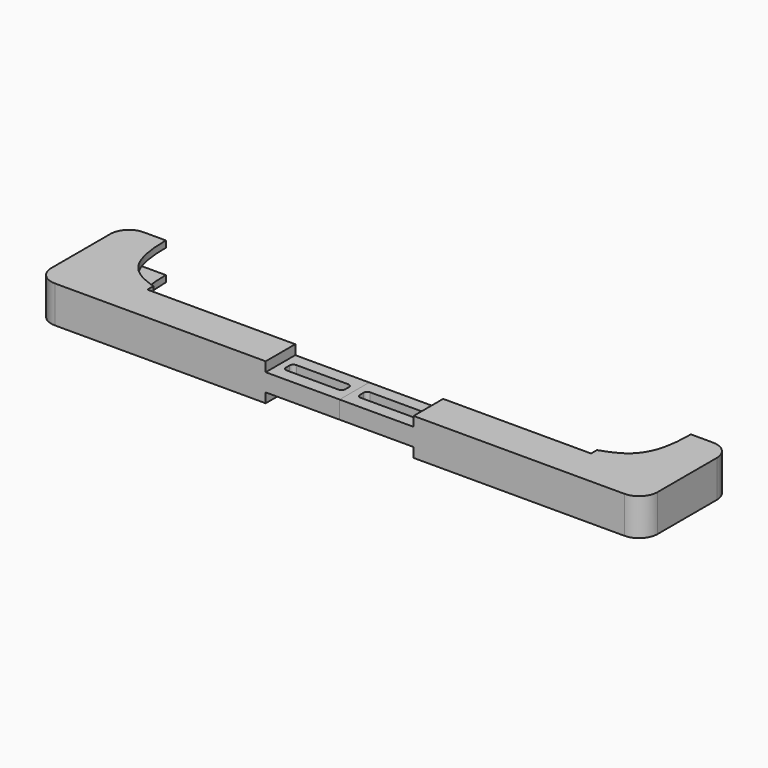
from build123d import *

# Parameters (mm, degrees)
F0_W         = 22
F0_H         = 30
F1_DEPTH     = 5
F2_W         = 18
F2_H         = 6.5
F3_DEPTH     = 18
F4_W         = 10
F4_H         = 10
F5_DEPTH     = 40
F6_W         = 10
F6_H         = 4.8
F7_DEPTH     = 20
F9_DEPTH     = 4.8
F11_DEPTH    = 10
F12_R        = 5
F13_T1_DEPTH = 35


# Not quite as in the source:
# - a fillet or chamfer that OpenCascade refuses, or shapes differently, is made with other operations: its cross-section is extruded or revolved along the edge and cut away or added


with BuildPart() as f1:
    # F0 (on Top) → F1 (new body, symmetric)
    with BuildSketch(Plane.XY):
        Rectangle(F0_W, F0_H)
    extrude(amount=F1_DEPTH, both=True)

    # F2 (on face) → F3 (cut)
    with BuildSketch(Plane(origin=(0, 15, 0), x_dir=(-1, 0, 0), z_dir=(0, 1, 0))):
        with Locations((2, 0)):
            Rectangle(F2_W, F2_H)
    extrude(amount=-F3_DEPTH, mode=Mode.SUBTRACT)

    # F4 (on face) → F5 (join)
    with BuildSketch(Plane(origin=(-11, 0, 0), x_dir=(0, -1, 0), z_dir=(-1, 0, 0))):
        with Locations((10, 0)):
            Rectangle(F4_W, F4_H)
    extrude(amount=F5_DEPTH)

    # F6 (on face) → F7 (join)
    with BuildSketch(Plane(origin=(-51, 0, 0), x_dir=(0, -1, 0), z_dir=(-1, 0, 0))):
        with Locations((10, 0)):
            Rectangle(F6_W, F6_H)
    extrude(amount=F7_DEPTH)

    # F8 (on face) → F9 (cut, through all)
    with BuildSketch(Plane.XY.offset(2.4)):
        with BuildLine():
            Line((-54, -8.4), (-68, -8.4))
            ThreePointArc((-68, -8.4), (-68.7071067812, -8.6928932188), (-69, -9.4))
            Line((-69, -9.4), (-69, -10.6))
            ThreePointArc((-69, -10.6), (-68.7071067812, -11.3071067812), (-68, -11.6))
            Line((-68, -11.6), (-54, -11.6))
            ThreePointArc((-54, -11.6), (-53.2928932188, -11.3071067812), (-53, -10.6))
            Line((-53, -10.6), (-53, -9.4))
            ThreePointArc((-53, -9.4), (-53.2928932188, -8.6928932188), (-54, -8.4))
        make_face()
    extrude(amount=-F9_DEPTH, mode=Mode.SUBTRACT)

    # F10 (on face) → F11 (cut, through all)
    with BuildSketch(Plane.XY.offset(5)):
        with BuildLine():
            add(Edge.make_bspline(
                [(0, 15), (0, 6.0453137533), (-3.1729094877, -0.7953640379), (-10.9956707869, -2.9450245736), (-11, -3)],
                knots=[0, 0, 0, 0, 0.6345947949, 1, 1, 1, 1], degree=3))
            Line((0, 15), (-11, 15))
            Line((-11, 15), (-11, -3))
        make_face()
    extrude(amount=-F11_DEPTH, mode=Mode.SUBTRACT)

    # F12
    f12_edges = [f1.edges().sort_by_distance(p)[0] for p in [
        (11, -15, 0),
    ]]
    fillet(f12_edges, radius=F12_R)

    # F13: fillet of radius 5 on 1 edges, made by hand

    # F13_s2 → F13_t1 (cut)
    with BuildSketch(Plane.XY.offset(-17.5)):
        with BuildLine():
            ThreePointArc((11, 10), (9.5355339059, 13.5355339059), (6, 15))
            Line((6, 15), (11, 15))
            Line((11, 15), (11, 10))
        make_face()
    extrude(amount=F13_T1_DEPTH, mode=Mode.SUBTRACT)


with BuildPart() as f14_1:
    # F14: instance of F1
    add(f1.part.mirror(Plane(origin=(-71, -10, 0), x_dir=(0, -1, 0), z_dir=(-1, 0, 0))))


solid = Compound([f1.part, f14_1.part])
